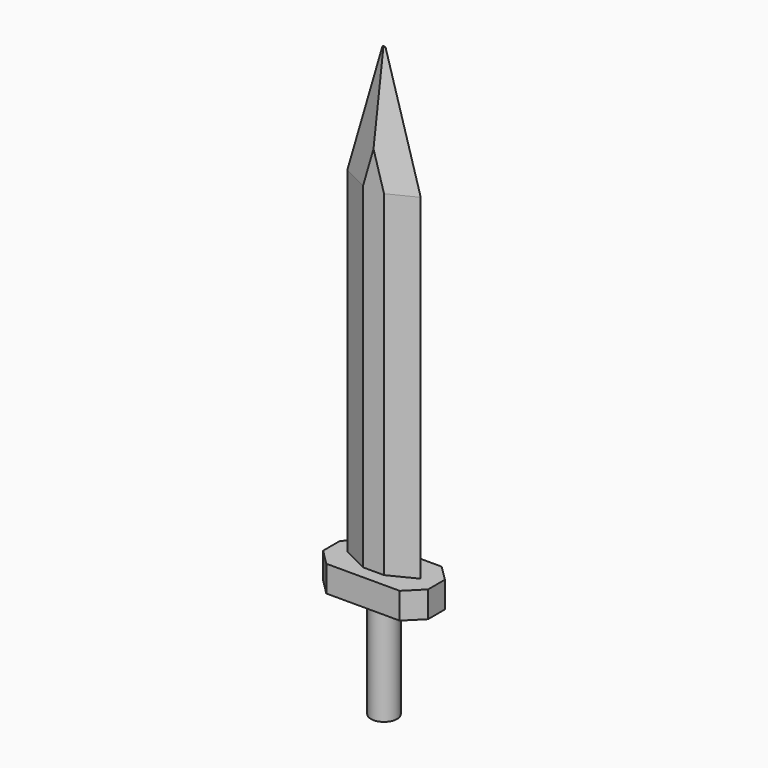
from build123d import *

# Parameters (mm, degrees)
F0_W        = 50.8
F0_H        = 25.4
F1_DEPTH    = 12.7
F2_R        = 6.35
F3_DEPTH    = 50.8
F4_W        = 35.56
F4_H        = 12.7
F5_DEPTH    = 220.98
F6_SIZE2    = 12.69999
F6_SIZE     = 6.34999
F6_2_SIZE2  = 12.69999
F6_2_SIZE   = 6.34999
F7_T1_DEPTH = 317.8886374297
F7_T3_DEPTH = 317.8886374297
F7_T5_DEPTH = 317.8886374297
F7_T7_DEPTH = 317.8886374297
F8_SIZE2    = 7.62
F8_SIZE     = 7.62


# Not quite as in the source:
# - a fillet or chamfer that OpenCascade refuses, or shapes differently, is made with other operations: its cross-section is extruded or revolved along the edge and cut away or added
# - a fillet or chamfer is up to 0.001 mm smaller than in the source, because OpenCascade refuses the exact size


with BuildPart() as f1:
    # F0 (on Top) → F1 (new body)
    with BuildSketch(Plane.XY):
        Rectangle(F0_W, F0_H)
    extrude(amount=F1_DEPTH)

    # F2 (on face) → F3 (join)
    with BuildSketch(Plane(origin=(0, 0, 0), x_dir=(1, 0, 0), z_dir=(0, 0, -1))):
        Circle(F2_R)
    extrude(amount=F3_DEPTH)

    # F4 (on face) → F5 (join)
    with BuildSketch(Plane.XY.offset(12.7)):
        Rectangle(F4_W, F4_H)
    extrude(amount=F5_DEPTH)

    # F6 (size 6.35 and 12.7 in the source; OpenCascade refuses exactly that, so slightly less here)
    f6_edges = [f1.edges().sort_by_distance(p)[0] for p in [
        (17.78, -6.35, 123.19),
        (17.78, 6.35, 123.19),
    ]]
    f6_side = f1.faces().sort_by_distance((17.78, 0, 123.19))[0]
    chamfer(f6_edges, length=F6_SIZE, length2=F6_SIZE2, reference=f6_side)

    # F6#2 (size 6.35 and 12.7 in the source; OpenCascade refuses exactly that, so slightly less here)
    f6_2_edges = [f1.edges().sort_by_distance(p)[0] for p in [
        (-17.78, 6.35, 123.19),
        (-17.78, -6.35, 123.19),
    ]]
    f6_2_side = f1.faces().sort_by_distance((-17.78, 0, 123.19))[0]
    chamfer(f6_2_edges, length=F6_2_SIZE, length2=F6_2_SIZE2, reference=f6_2_side)

    # F7: chamfer of 7.62 x 58.42 on 4 edges, made by hand

    # F7_s2 → F7_t1 (cut)
    with BuildSketch(Plane(origin=(150.0381483816, -75.0190151206, 0), x_dir=(0, 0, 1), z_dir=(-0.8944273319, 0.4472133138, 0))):
        Polygon((175.26, 7.9514616635), (233.68, 0.3314616635), (233.68, 7.9514616635), align=None)
    extrude(amount=F7_T1_DEPTH, mode=Mode.SUBTRACT)

    # F7_s4 → F7_t3 (cut)
    with BuildSketch(Plane(origin=(150.0381483816, 75.0190151206, 0), x_dir=(0, 0, 1), z_dir=(-0.8944273319, -0.4472133138, 0))):
        Polygon((175.26, -7.9514616635), (233.68, -0.3314616635), (233.68, -7.9514616635), align=None)
    extrude(amount=F7_T3_DEPTH, mode=Mode.SUBTRACT)

    # F7_s6 → F7_t5 (cut)
    with BuildSketch(Plane(origin=(-150.0381483816, 75.0190151206, 0), x_dir=(0, 0, 1), z_dir=(0.8944273319, -0.4472133138, 0))):
        Polygon((175.26, 7.9514616635), (233.68, 0.3314616635), (233.68, 7.9514616635), align=None)
    extrude(amount=F7_T5_DEPTH, mode=Mode.SUBTRACT)

    # F7_s8 → F7_t7 (cut)
    with BuildSketch(Plane(origin=(-150.0381483816, -75.0190151206, 0), x_dir=(0, 0, 1), z_dir=(0.8944273319, 0.4472133138, 0))):
        Polygon((175.26, -7.9514616635), (233.68, -0.3314616635), (233.68, -7.9514616635), align=None)
    extrude(amount=F7_T7_DEPTH, mode=Mode.SUBTRACT)

    # F8
    f8_edges = [f1.edges().sort_by_distance(p)[0] for p in [
        (-25.4, -12.7, 6.35),
        (25.4, -12.7, 6.35),
        (25.4, 12.7, 6.35),
        (-25.4, 12.7, 6.35),
    ]]
    chamfer(f8_edges, length=F8_SIZE, length2=F8_SIZE2)


solid = f1.part
